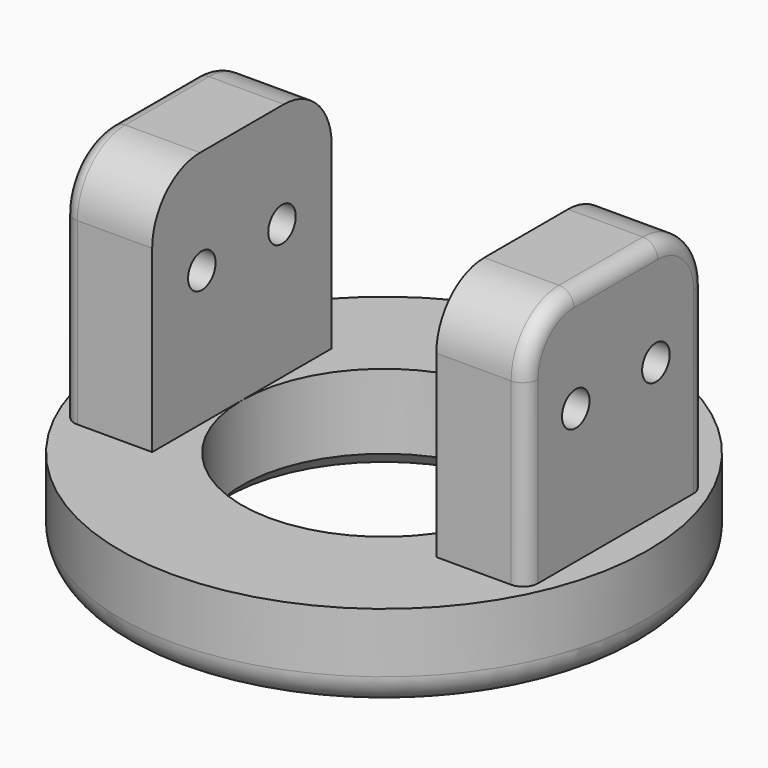
from build123d import *

# Parameters (mm, degrees)
F0_R     = 22.4155
F1_DEPTH = 7.62
F2_R     = 12.065
F3_DEPTH = 25.4
F5_DEPTH = 20.32
F6_R     = 5.08
F7_R     = 1.27
F8_R     = 1.4605
F9_DEPTH = 76.2
F11_SIZE = 1.27


# Not quite as in the source:
# - a fillet or chamfer that OpenCascade refuses, or shapes differently, is made with other operations: its cross-section is extruded or revolved along the edge and cut away or added


with BuildPart() as f1:
    # F0 (on Top) → F1 (new body)
    with BuildSketch(Plane.XY):
        with Locations((-27.5733582675, -25.1242369413)):
            Circle(F0_R)
    extrude(amount=F1_DEPTH)

    # F2 (on face) → F3 (cut)
    with BuildSketch(Plane.XY.offset(7.62)):
        with BuildLine():
            add(Edge.make_bspline(
                [(-22.4933582675, -7.3442369413), (-22.4933582675, -2.7248574376), (-30.1133582675, -5.0345471894), (-37.7333582675, -7.3442369413), (-30.1133582675, -9.6539266932), (-22.4933582675, -11.9636164451), (-22.4933582675, -7.3442369413)],
                knots=[0, 0, 0, 2.0943951024, 2.0943951024, 4.1887902048, 4.1887902048, 6.2831853072, 6.2831853072, 6.2831853072], degree=2, weights=[1, 0.5, 1, 0.5, 1, 0.5, 1]))
        make_face()
        with Locations((-27.5733582675, -25.1242369413)):
            Circle(F2_R)
    extrude(amount=-F3_DEPTH, mode=Mode.SUBTRACT)

    # F4 (on face) → F5 (join)
    with BuildSketch(Plane.XY.offset(7.62)):
        Polygon((-39.6383582675, -34.6492369413), (-39.6383582675, -25.1242369413), (-39.6383582675, -15.5992369413), (-47.2583582675, -15.5992369413), (-47.2583582675, -34.6492369413), align=None)
        Polygon((-7.8883582675, -34.6492369413), (-7.8883582675, -15.5992369413), (-15.5083582675, -15.5992369413), (-15.5083582675, -25.1242369413), (-15.5083582675, -34.6492369413), align=None)
    extrude(amount=F5_DEPTH)

    # F6
    f6_edges = [f1.edges().sort_by_distance(p)[0] for p in [
        (-11.698358, -34.649237, 27.94),
        (-11.698358, -15.599237, 27.94),
        (-43.448358, -34.649237, 27.94),
        (-43.448358, -15.599237, 27.94),
    ]]
    fillet(f6_edges, radius=F6_R)

    # F7
    f7_edges = [f1.edges().sort_by_distance(p)[0] for p in [
        (-7.888358, -34.649237, 15.24),
        (-47.258358, -15.599237, 15.24),
        (-47.258358, -34.649237, 15.24),
        (-47.258358, -33.161339, 26.452102),
        (-47.258358, -25.124237, 27.94),
        (-47.258358, -17.087134, 26.452102),
        (-7.888358, -33.161339, 26.452102),
        (-7.888358, -25.124237, 27.94),
        (-7.888358, -15.599237, 15.24),
        (-7.888358, -17.087134, 26.452102),
    ]]
    fillet(f7_edges, radius=F7_R)

    # F8 (on face) → F9 (cut)
    with BuildSketch(Plane(origin=(-47.2583582675, 0, 0), x_dir=(0, -1, 0), z_dir=(-1, 0, 0))):
        with Locations((20.8697369413, 19.05)):
            Circle(F8_R)
        with Locations((29.3787369413, 19.05)):
            Circle(F8_R)
    extrude(amount=-F9_DEPTH, mode=Mode.SUBTRACT)

    # F10: fillet of radius 2.54 on 1 edges, made by hand

    # F10_s1 → F10_t2 (revolve, cut)
    with BuildSketch(Plane.XZ.offset(25.1242369413)):
        with BuildLine():
            ThreePointArc((-5.1578582675, 2.54), (-5.9018070433, 0.7439487758), (-7.6978582675, 0))
            Line((-7.6978582675, 0), (-7.6978582675, -0.0508))
            Line((-7.6978582675, -0.0508), (-5.1070582675, -0.0508))
            Line((-5.1070582675, -0.0508), (-5.1070582675, 2.54))
            Line((-5.1070582675, 2.54), (-5.1578582675, 2.54))
        make_face()
    revolve(axis=Axis((-27.5733582675, -25.1242369413, 0), (0, 0, 1)), mode=Mode.SUBTRACT)

    # F11
    f11_edges = [f1.edges().sort_by_distance(p)[0] for p in [
        (-39.638358, -25.124237, 0),
    ]]
    chamfer(f11_edges, length=F11_SIZE)


solid = f1.part
